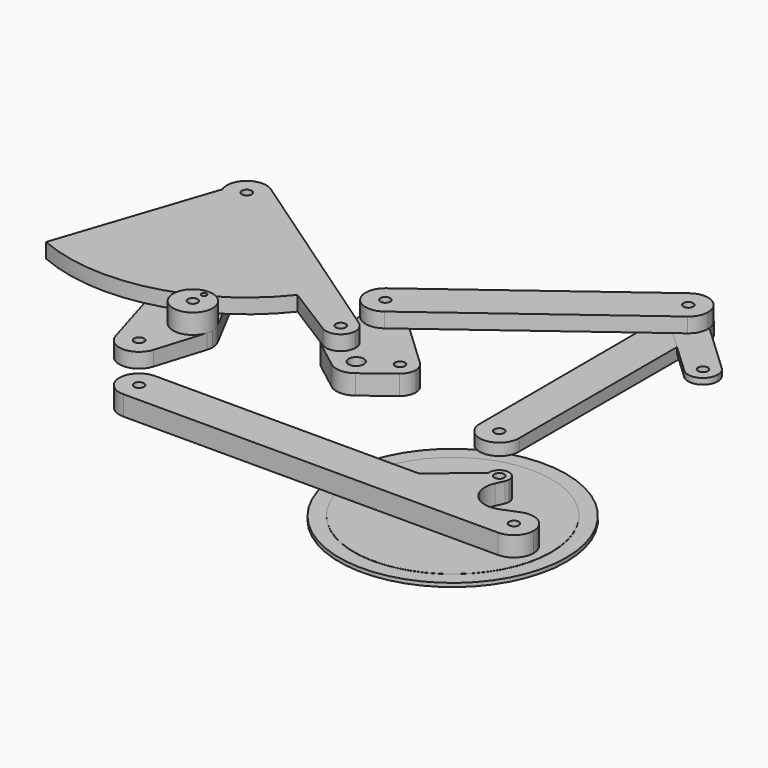
from build123d import *

# Parameters (mm, degrees)
F1_R      = 6.35
F2_DEPTH  = 19.05
F3_R      = 6.35
F3_R_2    = 15.24
F4_DEPTH  = 19.05
F5_R      = 25.4
F5_R_2    = 3.391909558
F5_R_3    = 6.35
F6_DEPTH  = 25.4
F7_R      = 6.35
F7_R_2    = 9.8146033801
F8_DEPTH  = 25.4
F10_R     = 6.35
F11_DEPTH = 25.4
F12_R     = 6.35
F13_DEPTH = 19.05
F14_R     = 6.35
F15_DEPTH = 15.24
F16_R     = 6.35
F17_DEPTH = 7.62
F19_R     = 146.05
F19_R_2   = 127
F20_DEPTH = 4.7752
F21_DEPTH = 0.254


# Not quite as in the source:
# - ends of sketch curves that miss each other by under 0.0002 mm in the source are joined


with BuildPart() as f2:
    # F1 (on Top) → F2 (new body)
    with BuildSketch(Plane.XY):
        with BuildLine():
            ThreePointArc((-348.2908615979, 65.3752063053), (-322.5061251941, 64.6802886665), (-309.4089688568, 86.90190062))
            ThreePointArc((-309.4089688568, 86.90190062), (-312.3358705821, 98.7391238559), (-320.4420282219, 107.848284957))
            ThreePointArc((-320.4420282219, 107.848284957), (-350.787985368, 106.6460397842), (-358.2902966075, 77.2175190155))
            ThreePointArc((-358.2902966075, 77.2175190155), (-354.2159266262, 70.5150159211), (-348.2908615979, 65.3752063053))
        make_face()
        with Locations((-334.8089688568, 86.90190062)):
            Circle(F1_R, mode=Mode.SUBTRACT)
        with BuildLine():
            ThreePointArc((-320.4420282219, 107.848284957), (-312.3358705821, 98.7391238559), (-309.4089688568, 86.90190062))
            ThreePointArc((-309.4089688568, 86.90190062), (-322.5061251941, 64.6802886665), (-348.2908615979, 65.3752063053))
            Line((-348.2908615979, 65.3752063053), (-155.7502543241, -55.2105082327))
            ThreePointArc((-155.7502543241, -55.2105082327), (-143.6386238017, -38.4450545545), (-133.0918711804, -20.6535385963))
            Line((-133.0918711804, -20.6535385963), (-320.4420282219, 107.848284957))
        make_face()
        with BuildLine():
            Line((-69.1399699738, -64.5175846932), (-133.0918711804, -20.6535385963))
            ThreePointArc((-133.0918711804, -20.6535385963), (-143.6386238017, -38.4450545545), (-155.7502543241, -55.2105082327))
            Line((-155.7502543241, -55.2105082327), (-90.0265950058, -96.372393682))
            ThreePointArc((-90.0265950058, -96.372393682), (-95.8460375379, -69.7817933481), (-69.1399699738, -64.5175846932))
        make_face()
        with BuildLine():
            ThreePointArc((-60.86517545, -80.227372946), (-63.060351744, -71.3494555191), (-69.1399699738, -64.5175846932))
            ThreePointArc((-69.1399699738, -64.5175846932), (-95.8460375379, -69.7817933481), (-90.0265950058, -96.372393682))
            ThreePointArc((-90.0265950058, -96.372393682), (-70.688042703, -96.8935819111), (-60.86517545, -80.227372946))
        make_face()
        with Locations((-79.91517545, -80.227372946)):
            Circle(F1_R, mode=Mode.SUBTRACT)
        with BuildLine():
            Line((-155.7502543241, -55.2105082327), (-348.2908615979, 65.3752063053))
            ThreePointArc((-348.2908615979, 65.3752063053), (-354.2159266262, 70.5150159211), (-358.2902966075, 77.2175190155))
            Line((-358.2902966075, 77.2175190155), (-425.0552400863, -123.1304076784))
            ThreePointArc((-425.0552400863, -123.1304076784), (-278.9055637141, -134.7572279839), (-155.7502543241, -55.2105082327))
        make_face()
    extrude(amount=F2_DEPTH)


with BuildPart() as f4:
    # F3 (on Top) → F4 (new body)
    with BuildSketch(Plane.XY):
        with BuildLine():
            ThreePointArc((-353.0581589295, 81.4365953504), (-332.0471371173, 68.0531663006), (-315.7589688568, 86.90190062))
            ThreePointArc((-315.7589688568, 86.90190062), (-316.3165540739, 91.4771706117), (-317.9566691714, 95.7846082767))
            ThreePointArc((-317.9566691714, 95.7846082767), (-342.0168946626, 104.5356269868), (-353.0581589295, 81.4365953504))
        make_face()
        with Locations((-334.8089688568, 86.90190062)):
            Circle(F3_R, mode=Mode.SUBTRACT)
        with BuildLine():
            ThreePointArc((-317.9566691714, 95.7846082767), (-316.3165540739, 91.4771706117), (-315.7589688568, 86.90190062))
            ThreePointArc((-315.7589688568, 86.90190062), (-332.0471371173, 68.0531663006), (-353.0581589295, 81.4365953504))
            Line((-353.0581589295, 81.4365953504), (-265.6322534303, -210.4870736928))
            ThreePointArc((-265.6322534303, -210.4870736928), (-244.9824423193, -178.0683542408), (-215.9, -203.2))
            ThreePointArc((-215.9, -203.2), (-216.1834122755, -206.9837839628), (-217.0273244943, -210.6831292782))
            Line((-217.0273244943, -210.6831292782), (-197.7546415567, -148.1692314583))
            ThreePointArc((-197.7546415567, -148.1692314583), (-247.3175108343, -143.0453603229), (-199.5575841486, -128.8424919711))
            Line((-199.5575841486, -128.8424919711), (-317.9566691714, 95.7846082767))
        make_face()
        with BuildLine():
            ThreePointArc((-196.6273170625, -140.6861021801), (-197.3707640186, -134.5857421912), (-199.5575841486, -128.8424919711))
            ThreePointArc((-199.5575841486, -128.8424919711), (-247.3175108343, -143.0453603229), (-197.7546415567, -148.1692314583))
            ThreePointArc((-197.7546415567, -148.1692314583), (-196.9107293379, -144.4698861429), (-196.6273170625, -140.6861021801))
        make_face()
        with Locations((-222.0273170625, -140.6861021801)):
            Circle(F3_R_2, mode=Mode.SUBTRACT)
        with BuildLine():
            ThreePointArc((-215.9, -203.2), (-244.9824423193, -178.0683542408), (-265.6322534303, -210.4870736928))
            ThreePointArc((-265.6322534303, -210.4870736928), (-241.4024540405, -228.5997933686), (-217.0273244943, -210.6831292782))
            ThreePointArc((-217.0273244943, -210.6831292782), (-216.1834122755, -206.9837839628), (-215.9, -203.2))
        make_face()
        with Locations((-241.3, -203.2)):
            Circle(F3_R, mode=Mode.SUBTRACT)
    extrude(amount=-F4_DEPTH)


with BuildPart() as f6:
    # F5 (on Top) → F6 (new body)
    with BuildSketch(Plane.XY):
        with Locations((-222.0273170625, -140.6861021801)):
            Circle(F5_R)
        with Locations((-222.0273170625, -122.6615665425)):
            Circle(F5_R_2, mode=Mode.SUBTRACT)
        with Locations((-222.0273170625, -140.6861021801)):
            Circle(F5_R_3, mode=Mode.SUBTRACT)
    extrude(amount=F6_DEPTH)


with BuildPart() as f8:
    # F7 (on Top) → F8 (new body)
    with BuildSketch(Plane.XY):
        with BuildLine():
            ThreePointArc((-100.23517545, -8.5105931449), (-79.91517545, -28.8305931449), (-59.59517545, -8.5105931449))
            ThreePointArc((-59.59517545, -8.5105931449), (-61.2619007451, -0.4509565039), (-65.9886540706, 6.2865147573))
            ThreePointArc((-65.9886540706, 6.2865147573), (-87.974812091, 10.14268156), (-100.23517545, -8.5105931449))
        make_face()
        with Locations((-79.91517545, -8.5105931449)):
            Circle(F7_R, mode=Mode.SUBTRACT)
        with BuildLine():
            ThreePointArc((-65.9886540706, 6.2865147573), (-61.2619007451, -0.4509565039), (-59.59517545, -8.5105931449))
            ThreePointArc((-59.59517545, -8.5105931449), (-79.91517545, -28.8305931449), (-100.23517545, -8.5105931449))
            Line((-100.23517545, -8.5105931449), (-100.23517545, -80.227372946))
            ThreePointArc((-100.23517545, -80.227372946), (-79.91517545, -59.907372946), (-59.59517545, -80.227372946))
            ThreePointArc((-59.59517545, -80.227372946), (-59.7853586301, -83.0009761617), (-60.3523481664, -85.7226608066))
            ThreePointArc((-60.3523481664, -85.7226608066), (-41.81517545, -77.687372946), (-23.2780027336, -85.7226608066))
            ThreePointArc((-23.2780027336, -85.7226608066), (-14.2454801707, -62.8487918045), (10.2113459294, -65.4302650438))
            Line((10.2113459294, -65.4302650438), (-65.9886540706, 6.2865147573))
        make_face()
        with BuildLine():
            ThreePointArc((-65.8603556748, -94.9026733207), (-78.8102903137, -100.5173120498), (-92.2933308728, -96.3420764285))
            Line((-92.2933308728, -96.3420764285), (-57.2878697285, -123.2307522991))
            ThreePointArc((-57.2878697285, -123.2307522991), (-66.1263995238, -110.4443005678), (-65.8603556748, -94.9026733207))
        make_face()
        with BuildLine():
            ThreePointArc((-59.59517545, -80.227372946), (-79.91517545, -59.907372946), (-100.23517545, -80.227372946))
            ThreePointArc((-100.23517545, -80.227372946), (-98.1418937255, -89.2100863948), (-92.2933308728, -96.3420764285))
            ThreePointArc((-92.2933308728, -96.3420764285), (-78.8102903137, -100.5173120498), (-65.8603556748, -94.9026733207))
            ThreePointArc((-65.8603556748, -94.9026733207), (-63.5954957631, -90.0191807581), (-60.3523481664, -85.7226608066))
            ThreePointArc((-60.3523481664, -85.7226608066), (-59.7853586301, -83.0009761617), (-59.59517545, -80.227372946))
        make_face()
        with Locations((-79.91517545, -80.227372946)):
            Circle(F7_R, mode=Mode.SUBTRACT)
        with BuildLine():
            ThreePointArc((-17.7699952252, -94.9026733207), (-21.1394317005, -90.6819266963), (-23.2780027336, -85.7226608066))
            ThreePointArc((-23.2780027336, -85.7226608066), (-41.81517545, -77.687372946), (-60.3523481664, -85.7226608066))
            ThreePointArc((-60.3523481664, -85.7226608066), (-62.4909191995, -90.6819266963), (-65.8603556748, -94.9026733207))
            ThreePointArc((-65.8603556748, -94.9026733207), (-66.1263995238, -110.4443005678), (-57.2878697285, -123.2307522991))
            ThreePointArc((-57.2878697285, -123.2307522991), (-41.81517545, -128.487372946), (-26.3424811715, -123.2307522991))
            ThreePointArc((-26.3424811715, -123.2307522991), (-19.0317776056, -114.3157647571), (-16.41517545, -103.087372946))
            ThreePointArc((-16.41517545, -103.087372946), (-16.7561693074, -98.9393359229), (-17.7699952252, -94.9026733207))
        make_face()
        with Locations((-41.81517545, -103.087372946)):
            Circle(F7_R_2, mode=Mode.SUBTRACT)
        with BuildLine():
            ThreePointArc((-65.8603556748, -94.9026733207), (-62.4909191995, -90.6819266963), (-60.3523481664, -85.7226608066))
            ThreePointArc((-60.3523481664, -85.7226608066), (-63.5954957631, -90.0191807581), (-65.8603556748, -94.9026733207))
        make_face()
        with BuildLine():
            ThreePointArc((-17.7699952252, -94.9026733207), (-20.0348551369, -90.0191807581), (-23.2780027336, -85.7226608066))
            ThreePointArc((-23.2780027336, -85.7226608066), (-21.1394317005, -90.6819266963), (-17.7699952252, -94.9026733207))
        make_face()
        with BuildLine():
            ThreePointArc((16.60482455, -80.227372946), (14.9380992549, -72.167736305), (10.2113459294, -65.4302650438))
            ThreePointArc((10.2113459294, -65.4302650438), (-14.2454801707, -62.8487918045), (-23.2780027336, -85.7226608066))
            ThreePointArc((-23.2780027336, -85.7226608066), (-20.0348551369, -90.0191807581), (-17.7699952252, -94.9026733207))
            ThreePointArc((-17.7699952252, -94.9026733207), (-4.8200605863, -100.5173120498), (8.6629799728, -96.3420764285))
            ThreePointArc((8.6629799728, -96.3420764285), (14.5115428255, -89.2100863948), (16.60482455, -80.227372946))
        make_face()
        with Locations((-3.71517545, -80.227372946)):
            Circle(F7_R, mode=Mode.SUBTRACT)
        with BuildLine():
            Line((-26.3424811715, -123.2307522991), (8.6629799728, -96.3420764285))
            ThreePointArc((8.6629799728, -96.3420764285), (-4.8200605863, -100.5173120498), (-17.7699952252, -94.9026733207))
            ThreePointArc((-17.7699952252, -94.9026733207), (-16.7561693074, -98.9393359229), (-16.41517545, -103.087372946))
            ThreePointArc((-16.41517545, -103.087372946), (-19.0317776056, -114.3157647571), (-26.3424811715, -123.2307522991))
        make_face()
    extrude(amount=-F8_DEPTH)


with BuildPart() as f11:
    # F10 (on offset) → F11 (new body)
    with BuildSketch(Plane.XY.offset(-50.8)):
        with BuildLine():
            ThreePointArc((-241.3, -228.6), (-223.3394877579, -221.1605122421), (-215.9, -203.2))
            ThreePointArc((-215.9, -203.2), (-223.3394877579, -185.2394877579), (-241.3, -177.8))
            ThreePointArc((-241.3, -177.8), (-266.7, -203.2), (-241.3, -228.6))
        make_face()
        with Locations((-241.3, -203.2)):
            Circle(F10_R, mode=Mode.SUBTRACT)
        with BuildLine():
            ThreePointArc((-241.3, -177.8), (-223.3394877579, -185.2394877579), (-215.9, -203.2))
            ThreePointArc((-215.9, -203.2), (-223.3394877579, -221.1605122421), (-241.3, -228.6))
            Line((-241.3, -228.6), (241.3, -228.6))
            ThreePointArc((241.3, -228.6), (216.3562277503, -207.9925177054), (231.8871283349, -179.6085217289))
            Line((231.8871283349, -179.6085217289), (211.0097267055, -187.9384915587))
            ThreePointArc((211.0097267055, -187.9384915587), (177.641099394, -180.6478771481), (171.9905944387, -146.9627151196))
            Line((171.9905944387, -146.9627151196), (176.6515359453, -136.7607212463))
            ThreePointArc((176.6515359453, -136.7607212463), (163.11346164, -144.0268905287), (152.4830404112, -132.9331618302))
            Line((152.4830404112, -132.9331618302), (99.012824834, -177.8))
            Line((99.012824834, -177.8), (-241.3, -177.8))
        make_face()
        with BuildLine():
            ThreePointArc((177.8, -131.4832201989), (164.3738411943, -118.8039972973), (152.4830404112, -132.9331618302))
            ThreePointArc((152.4830404112, -132.9331618302), (163.11346164, -144.0268905287), (176.6515359453, -136.7607212463))
            ThreePointArc((176.6515359453, -136.7607212463), (177.5095629759, -134.1837288079), (177.8, -131.4832201989))
        make_face()
        with Locations((165.1, -131.4832201989)):
            Circle(F10_R, mode=Mode.SUBTRACT)
        with BuildLine():
            ThreePointArc((231.8871283349, -179.6085217289), (216.3562277503, -207.9925177054), (241.3, -228.6))
            ThreePointArc((241.3, -228.6), (259.2605122421, -221.1605122421), (266.7, -203.2))
            ThreePointArc((266.7, -203.2), (255.5490887376, -182.1732677254), (231.8871283349, -179.6085217289))
        make_face()
        with Locations((241.3, -203.2)):
            Circle(F10_R, mode=Mode.SUBTRACT)
    extrude(amount=-F11_DEPTH)


with BuildPart() as f13:
    # F12 (on Top) → F13 (new body)
    with BuildSketch(Plane.XY):
        with BuildLine():
            ThreePointArc((-64.7629150633, -28.8961028313), (-57.2212620169, -19.9187609684), (-54.51517545, -8.5105931449))
            ThreePointArc((-54.51517545, -8.5105931449), (-68.5070076265, 14.1833202883), (-95.0674358367, 11.8749165415))
            ThreePointArc((-95.0674358367, 11.8749165415), (-100.3006851364, -23.6628535316), (-64.7629150633, -28.8961028313))
        make_face()
        with Locations((-79.91517545, -8.5105931449)):
            Circle(F12_R, mode=Mode.SUBTRACT)
        with BuildLine():
            ThreePointArc((-95.0674358367, 11.8749165415), (-68.5070076265, 14.1833202883), (-54.51517545, -8.5105931449))
            ThreePointArc((-54.51517545, -8.5105931449), (-57.2212620169, -19.9187609684), (-64.7629150633, -28.8961028313))
            Line((-64.7629150633, -28.8961028313), (179.8632011733, 152.9310218091))
            ThreePointArc((179.8632011733, 152.9310218091), (144.3254311003, 158.1642711088), (149.5586804, 193.7020411818))
            Line((149.5586804, 193.7020411818), (-95.0674358367, 11.8749165415))
        make_face()
        with BuildLine():
            ThreePointArc((190.1109407867, 173.3165314954), (176.1191086101, 196.0104449286), (149.5586804, 193.7020411818))
            ThreePointArc((149.5586804, 193.7020411818), (144.3254311003, 158.1642711088), (179.8632011733, 152.9310218091))
            ThreePointArc((179.8632011733, 152.9310218091), (187.4048542198, 161.908363672), (190.1109407867, 173.3165314954))
        make_face()
        with Locations((164.7109407867, 173.3165314954)):
            Circle(F12_R, mode=Mode.SUBTRACT)
    extrude(amount=F13_DEPTH)


with BuildPart() as f15:
    # F14 (on Top) → F15 (new body)
    with BuildSketch(Plane.XY):
        with BuildLine():
            ThreePointArc((190.3191387149, 173.312513352), (190.3191389513, 173.3145224237), (190.3191390301, 173.3165314954))
            ThreePointArc((190.3191390301, 173.3165314954), (164.6762443628, 198.9247062339), (139.1028365632, 173.2471387114))
            ThreePointArc((139.1028365632, 173.2471387114), (164.7436281405, 147.7083541137), (190.3191387149, 173.312513352))
        make_face()
        with Locations((164.7109407867, 173.3165314954)):
            Circle(F14_R, mode=Mode.SUBTRACT)
        with BuildLine():
            ThreePointArc((190.3191387149, 173.312513352), (164.7436281405, 147.7083541137), (139.1028365632, 173.2471387114))
            Line((139.1028365632, 173.2471387114), (139.9287790463, -131.5514291176))
            ThreePointArc((139.9287790463, -131.5514291176), (165.0658955093, -106.3119299332), (190.2713133697, -131.4832201989))
            Line((190.2713133697, -131.4832201989), (190.3191387149, 173.312513352))
        make_face()
        with BuildLine():
            ThreePointArc((190.2713133697, -131.4832201989), (165.0658955093, -106.3119299332), (139.9287790463, -131.5514291176))
            ThreePointArc((139.9287790463, -131.5514291176), (165.1321296961, -156.6545130627), (190.2713130598, -131.4871697914))
            ThreePointArc((190.2713130598, -131.4871697914), (190.2713132922, -131.4851949951), (190.2713133697, -131.4832201989))
        make_face()
        with Locations((165.1, -131.4832201989)):
            Circle(F14_R, mode=Mode.SUBTRACT)
    extrude(amount=-F15_DEPTH)


with BuildPart() as f17:
    # F16 (on Top) → F17 (new body)
    with BuildSketch(Plane.XY):
        with BuildLine():
            ThreePointArc((151.6548269934, 159.4442428372), (172.2668501376, 155.8290864596), (183.7609407867, 173.3165314954))
            ThreePointArc((183.7609407867, 173.3165314954), (182.1983858225, 180.8724408464), (177.7670545799, 187.1888201537))
            ThreePointArc((177.7670545799, 187.1888201537), (150.8386521284, 186.3726452887), (151.6548269934, 159.4442428372))
        make_face()
        with Locations((164.7109407867, 173.3165314954)):
            Circle(F16_R, mode=Mode.SUBTRACT)
        with BuildLine():
            ThreePointArc((177.7670545799, 187.1888201537), (182.1983858225, 180.8724408464), (183.7609407867, 173.3165314954))
            ThreePointArc((183.7609407867, 173.3165314954), (172.2668501376, 155.8290864596), (151.6548269934, 159.4442428372))
            Line((151.6548269934, 159.4442428372), (227.8548269934, 87.7274630361))
            ThreePointArc((227.8548269934, 87.7274630361), (227.0386521284, 114.6558654876), (253.9670545799, 115.4720403526))
            Line((253.9670545799, 115.4720403526), (177.7670545799, 187.1888201537))
        make_face()
        with BuildLine():
            ThreePointArc((259.9609407867, 101.5997516943), (258.3983858225, 109.1556610453), (253.9670545799, 115.4720403526))
            ThreePointArc((253.9670545799, 115.4720403526), (227.0386521284, 114.6558654876), (227.8548269934, 87.7274630361))
            ThreePointArc((227.8548269934, 87.7274630361), (248.4668501376, 84.1123066585), (259.9609407867, 101.5997516943))
        make_face()
        with Locations((240.9109407867, 101.5997516943)):
            Circle(F16_R, mode=Mode.SUBTRACT)
    extrude(amount=-F17_DEPTH)


with BuildPart() as f20:
    # F19 (on offset) → F20 (new body)
    with BuildSketch(Plane.XY.offset(-203.2)):
        Circle(F19_R)
        Circle(F19_R_2, mode=Mode.SUBTRACT)
        Circle(F19_R_2)
    extrude(amount=-F20_DEPTH)

    # F19 (on offset) → F21 (join)
    with BuildSketch(Plane.XY.offset(-203.2)):
        Circle(F19_R_2)
    extrude(amount=F21_DEPTH)


solid = Compound([f2.part, f4.part, f6.part, f8.part, f11.part, f13.part, f15.part, f17.part, f20.part])
